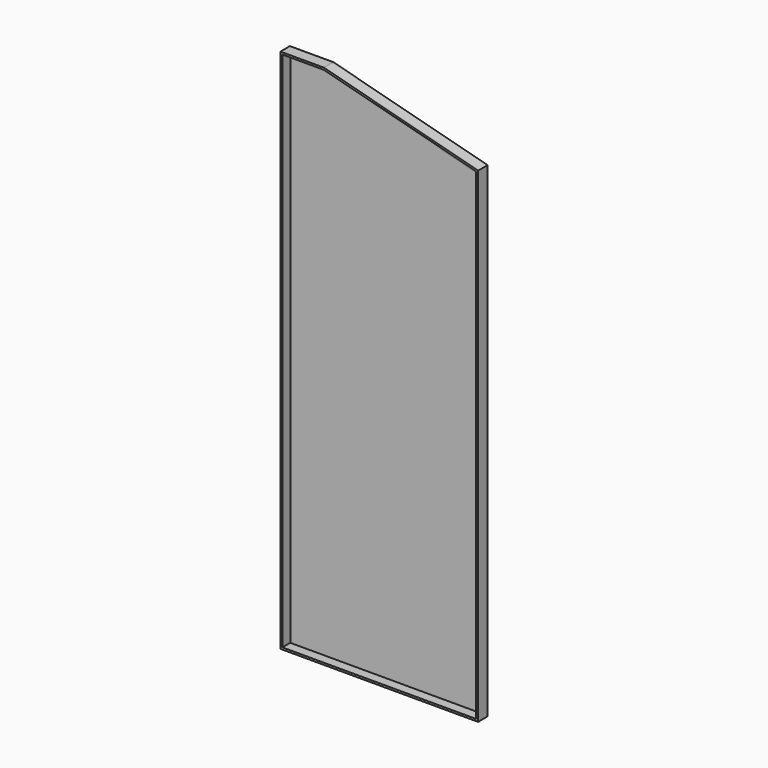
from build123d import *

# Parameters (mm, degrees)
F1_DEPTH = 6.35
F3_DEPTH = 31.75


# Not quite as in the source:
# - a length typed as a fraction of an inch, garbled in the dataset ("3 / 203.2 mm" for 3/8 in), is restored


with BuildPart() as f1:
    # F0 (on Front) → F1 (new body)
    with BuildSketch(Plane.XZ):
        Polygon((0, 1689.1), (0, 0), (635, 0), (635, 1558.925), (139.7, 1689.1), align=None)
    extrude(amount=-F1_DEPTH)

    # F2 (on Front) → F3 (join)
    with BuildSketch(Plane.XZ):
        Polygon((635, 0), (635, 1558.925), (139.7, 1689.1), (0, 1689.1), (0, 0), align=None)
        Polygon((6.35, 6.35), (6.35, 1682.75), (139.7, 1682.75), (628.65, 1554.2439102564), (628.65, 6.35), align=None, mode=Mode.SUBTRACT)
    extrude(amount=F3_DEPTH)


solid = f1.part
